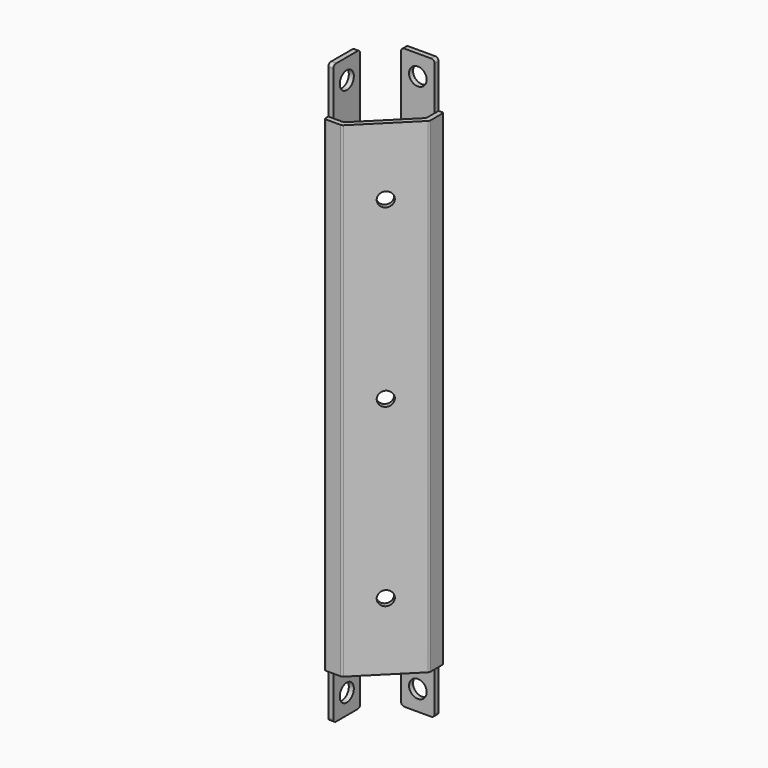
from build123d import *

# Parameters (mm, degrees)
F1_DEPTH = 172.5
F3_DEPTH = 28
F4_R     = 4.25
F5_DEPTH = 25
F6_R     = 5.25
F7_DEPTH = 25
F8_R     = 5.25
F9_DEPTH = 25
F10_R    = 2
F11_R    = 0.5
F12_R    = 1


# Not quite as in the source:
# - a pattern or mirror of a feature is missing from the dataset's text; its kind, count and spacing are read off the source's solid


with BuildPart() as f1:
    # F0 (on Top) → F1 (new body, symmetric)
    with BuildSketch(Plane.XY):
        Polygon((-19.75, 3.25), (-19.75, -19.75), (-9.25, -19.75), (19.75, 9.25), (19.75, 19.75), (-3.25, 19.75), (-3.25, 16.75), (16.75, 16.75), (16.75, 10.4926406871), (-10.4926406871, -16.75), (-16.75, -16.75), (-16.75, 3.25), align=None)
    extrude(amount=F1_DEPTH, both=True)

    # F2 (on face) → F3 (cut)
    with BuildSketch(Plane.XY.offset(172.5)):
        Polygon((-10.4926406871, -16.75), (-16.75, -16.75), (-19.75, -16.75), (-19.75, -19.75), (-9.25, -19.75), (19.75, 9.25), (19.75, 19.75), (16.75, 19.75), (16.75, 16.75), (16.75, 10.4926406871), align=None)
    f3 = extrude(amount=-F3_DEPTH, mode=Mode.SUBTRACT)

    # F3_copies: F3 across plane
    add(f3.mirror(Plane(origin=(0, 0, 0), x_dir=(-1, 0, 0), z_dir=(0, 0, -1))), mode=Mode.SUBTRACT)

    # F4 (on face) → F5 (cut)
    with BuildSketch(Plane(origin=(5.25, -5.25, 0), x_dir=(0.7071067812, 0.7071067812, 0), z_dir=(0.7071067812, -0.7071067812, 0))):
        with Locations((0, 104.5)):
            Circle(F4_R)
        with Locations((0, -104.5)):
            Circle(F4_R)
        Circle(F4_R)
    extrude(amount=-F5_DEPTH, mode=Mode.SUBTRACT)

    # F6 (on face) → F7 (cut)
    with BuildSketch(Plane.YZ.offset(-16.75)):
        with Locations((-6.75, 160.5)):
            Circle(F6_R)
        with Locations((-6.75, -160.5)):
            Circle(F6_R)
    extrude(amount=-F7_DEPTH, mode=Mode.SUBTRACT)

    # F8 (on face) → F9 (cut)
    with BuildSketch(Plane.XZ.offset(-16.75)):
        with Locations((6.75, 160.5)):
            Circle(F8_R)
        with Locations((6.75, -160.5)):
            Circle(F8_R)
    extrude(amount=-F9_DEPTH, mode=Mode.SUBTRACT)

    # F10
    f10_edges = [f1.edges().sort_by_distance(p)[0] for p in [
        (-9.25, -19.75, 0),
        (19.75, 9.25, 0),
        (16.75, 18.25, 172.5),
        (-3.25, 18.25, 172.5),
        (-18.25, 3.25, 172.5),
        (-18.25, -16.75, 172.5),
        (-18.25, 3.25, -172.5),
        (-3.25, 18.25, -172.5),
        (-18.25, -16.75, -172.5),
        (16.75, 18.25, -172.5),
    ]]
    fillet(f10_edges, radius=F10_R)

    # F11
    f11_edges = [f1.edges().sort_by_distance(p)[0] for p in [
        (-10.492641, -16.75, 0),
        (16.75, 10.492641, 0),
    ]]
    fillet(f11_edges, radius=F11_R)

    # F12
    f12_edges = [f1.edges().sort_by_distance(p)[0] for p in [
        (-19.75, -19.75, 0),
        (19.75, 19.75, 0),
    ]]
    fillet(f12_edges, radius=F12_R)


solid = f1.part
